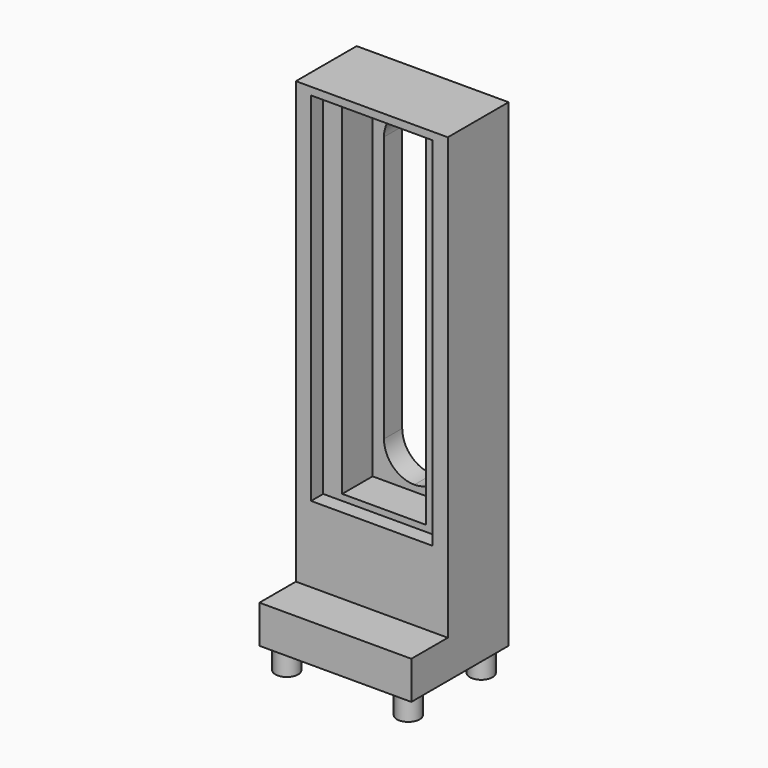
from build123d import *

# Parameters (mm, degrees)
F0_W     = 254
F0_H     = 736.6
F0_W_2   = 203.2
F0_H_2   = 596.9
F0_W_3   = 139.7
F0_H_3   = 571.5
F0_W_4   = 101.6
F0_H_4   = 546.1
F0_H_5   = 63.5
F1_DEPTH = 127
F2_DEPTH = 25.4
F3_DEPTH = 88.9
F4_R     = 50.79999
F5_DEPTH = 76.2
F6_R     = 19.05
F7_DEPTH = 38.1


# Not quite as in the source:
# - a fillet or chamfer is up to 0.001 mm smaller than in the source, because OpenCascade refuses the exact size
# - a feature names something its author has since deleted; it is built from what else it names


with BuildPart() as f1:
    # F0 (on Front) → F1 (new body)
    with BuildSketch(Plane.XZ):
        with Locations((0, 241.3)):
            Rectangle(F0_W, F0_H)
        with Locations((0, 298.45)):
            Rectangle(F0_W_2, F0_H_2, mode=Mode.SUBTRACT)
        with Locations((0, 298.45)):
            Rectangle(F0_W_2, F0_H_2)
        with Locations((0, 296.15)):
            Rectangle(F0_W_3, F0_H_3, mode=Mode.SUBTRACT)
        with Locations((0, 296.15)):
            Rectangle(F0_W_3, F0_H_3)
        with Locations((0, 293.85)):
            Rectangle(F0_W_4, F0_H_4, mode=Mode.SUBTRACT)
        with Locations((0, -158.75)):
            Rectangle(F0_W, F0_H_5)
    extrude(amount=-F1_DEPTH)

    # F0 (on Front) → F2 (cut)
    with BuildSketch(Plane.XZ):
        with Locations((0, 298.45)):
            Rectangle(F0_W_2, F0_H_2)
        with Locations((0, 296.15)):
            Rectangle(F0_W_3, F0_H_3, mode=Mode.SUBTRACT)
    extrude(amount=-F2_DEPTH, mode=Mode.SUBTRACT)

    # F0 (on Front) → F3 (cut)
    with BuildSketch(Plane.XZ):
        with Locations((0, 296.15)):
            Rectangle(F0_W_3, F0_H_3)
        with Locations((0, 293.85)):
            Rectangle(F0_W_4, F0_H_4, mode=Mode.SUBTRACT)
    extrude(amount=-F3_DEPTH, mode=Mode.SUBTRACT)

    # F4 (radius 50.8 in the source; OpenCascade refuses exactly that, so slightly less here)
    f4_edges = [f1.edges().sort_by_distance(p)[0] for p in [
        (50.8, 107.95, 566.9),
        (-50.8, 107.95, 566.9),
        (-50.8, 107.95, 20.8),
        (50.8, 107.95, 20.8),
    ]]
    fillet(f4_edges, radius=F4_R)

    # F0 (on Front) → F5 (join)
    with BuildSketch(Plane.XZ):
        with Locations((0, -158.75)):
            Rectangle(F0_W, F0_H_5)
    extrude(amount=F5_DEPTH)

    # F6 (on face) → F7 (join)
    with BuildSketch(Plane(origin=(0, 0, -190.5), x_dir=(1, 0, 0), z_dir=(0, 0, -1))):
        with Locations((-101.6, 50.8)):
            Circle(F6_R)
        with Locations((101.6, 50.8)):
            Circle(F6_R)
        with Locations((-101.6, -101.6)):
            Circle(F6_R)
        with Locations((101.6, -101.6)):
            Circle(F6_R)
    extrude(amount=F7_DEPTH)


solid = f1.part
